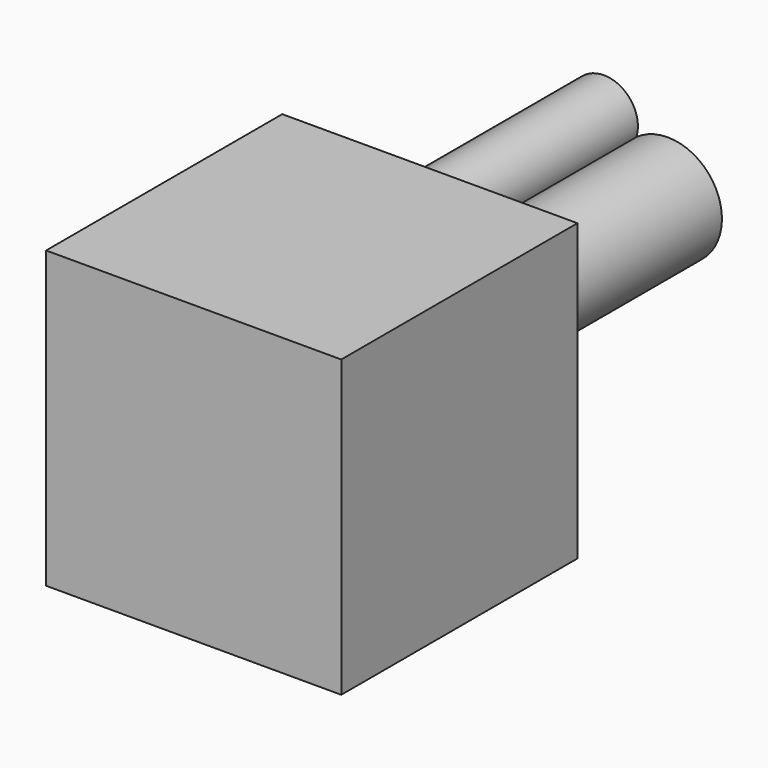
from build123d import *

# Parameters (mm, degrees)
F0_W     = 76.2
F0_H     = 76.2
F1_DEPTH = 76.2
F2_R     = 13.9945957695
F3_DEPTH = 76.2
F5_DEPTH = 76.2
F6_DEPTH = 0.127


# Not quite as in the source:
# - a feature of the source that left no trace in its solid (it failed there, or was rolled back) is left out


with BuildPart() as f1:
    # F0 (on Front) → F1 (new body)
    with BuildSketch(Plane.XZ):
        with Locations((-0.348880887, -0.3284779671)):
            Rectangle(F0_W, F0_H)
    extrude(amount=F1_DEPTH)

    # F2 (on face) → F3 (join)
    with BuildSketch(Plane(origin=(0, 0, 0), x_dir=(-1, 0, 0), z_dir=(0, 1, 0))):
        Circle(F2_R)
    extrude(amount=F3_DEPTH)

    # F4 (on face) → F5 (join)
    with BuildSketch(Plane(origin=(0, 0, 0), x_dir=(-1, 0, 0), z_dir=(0, 1, 0))):
        with BuildLine():
            ThreePointArc((12.5814202737, 6.1283419167), (21.0911235736, 6.5413963555), (25.2311478041, 13.9875942841))
            ThreePointArc((25.2311478041, 13.9875942841), (15.1695556684, 22.6577098126), (8.081240073, 11.4255096006))
            ThreePointArc((8.081240073, 11.4255096006), (10.6654291765, 9.0607577626), (12.5814202737, 6.1283419167))
        make_face()
        with BuildLine():
            ThreePointArc((13.1726915392, -4.7253474332), (11.363857458, -8.1677080277), (8.6776055388, -10.9794295328))
            ThreePointArc((8.6776055388, -10.9794295328), (16.220264771, -20.1665195025), (24.895431247, -12.0402770117))
            ThreePointArc((24.895431247, -12.0402770117), (21.0629315641, -5.1313910488), (13.1726915392, -4.7253474332))
        make_face()
        with BuildLine():
            ThreePointArc((13.1726915392, -4.7253474332), (10.1390684725, -7.2873978983), (8.6776055388, -10.9794295328))
            ThreePointArc((8.6776055388, -10.9794295328), (11.363857458, -8.1677080277), (13.1726915392, -4.7253474332))
        make_face()
    extrude(amount=F5_DEPTH)

    # F6 (add): a face of the model
    f6_faces = [f1.faces().sort_by_distance(p)[0] for p in [
        (-6.9646133447, 76.2, 0.8386205015),
    ]]
    extrude(f6_faces, amount=F6_DEPTH)


solid = f1.part
